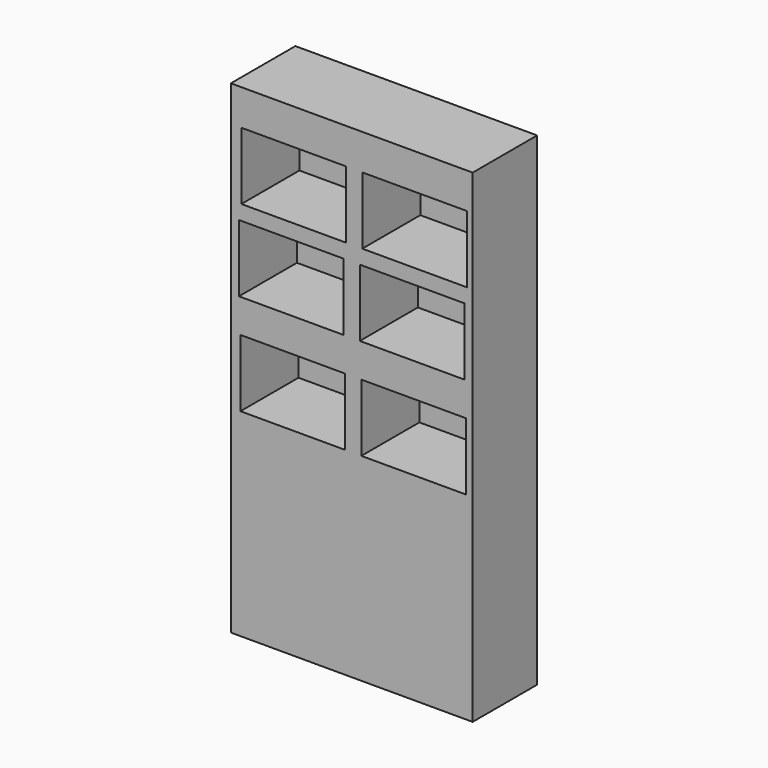
from build123d import *

# Parameters (mm, degrees)
F0_W     = 76.2
F0_H     = 152.4
F1_DEPTH = 25.4
F2_W     = 33.02
F2_H     = 21.1666666667
F3_DEPTH = 22.86
F4_DEPTH = 22.86
F5_DEPTH = 22.86


# Not quite as in the source:
# - a feature names something its author has since deleted; it is built from what else it names


with BuildPart() as f1:
    # F0 (on Front) → F1 (new body)
    with BuildSketch(Plane.XZ):
        Rectangle(F0_W, F0_H)
    extrude(amount=F1_DEPTH)

    # F2 (on face) → F3 (cut)
    with BuildSketch(Plane.XZ.offset(25.4)):
        with Locations((-18.2778849706, 54.3725310351)):
            Rectangle(F2_W, F2_H)
    extrude(amount=-F3_DEPTH, mode=Mode.SUBTRACT)

    # F2 (on face) → F4 (cut)
    with BuildSketch(Plane.XZ.offset(25.4)):
        with Locations((19.8221150294, 54.3725310351)):
            Rectangle(F2_W, F2_H)
        with Locations((-19.05, 28.5166088839)):
            Rectangle(F2_W, F2_H)
        with Locations((-18.5682759488, -3.211494873)):
            Rectangle(F2_W, F2_H)
        with Locations((19.5317240512, -3.211494873)):
            Rectangle(F2_W, F2_H)
    extrude(amount=-F4_DEPTH, mode=Mode.SUBTRACT)

    # F2 (on face) → F5 (cut)
    with BuildSketch(Plane.XZ.offset(25.4)):
        with Locations((19.05, 28.5166088839)):
            Rectangle(F2_W, F2_H)
    extrude(amount=-F5_DEPTH, mode=Mode.SUBTRACT)


solid = f1.part
